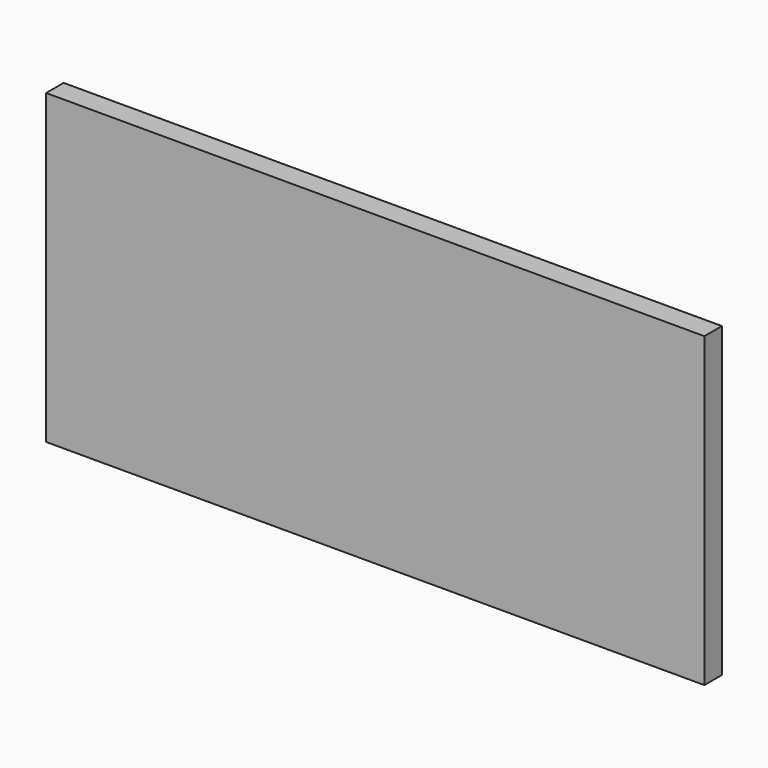
from build123d import *

# Parameters (mm, degrees)
F0_W     = 381
F0_H     = 177.8
F2_DEPTH = 12.7


# Not quite as in the source:
# - a variable given as a bare number and used for a length is read in inches; the dataset says mm whatever the document's units were


with BuildPart() as f2:
    # F0 (on Front) → F2 (new body)
    with BuildSketch(Plane.XZ):
        with Locations((190.5, -88.9)):
            Rectangle(F0_W, F0_H)
    extrude(amount=F2_DEPTH)


solid = f2.part
